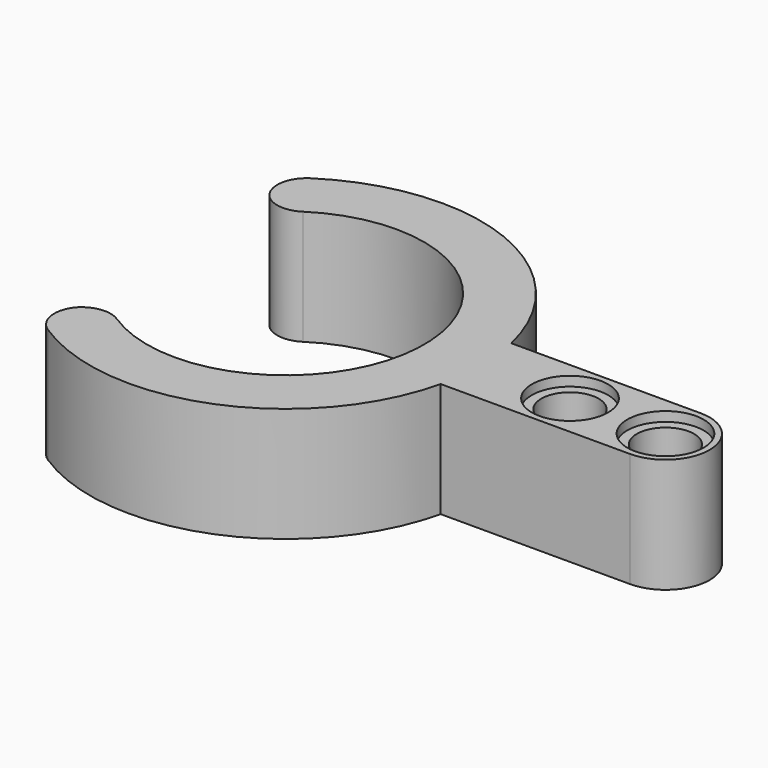
from build123d import *

# Parameters (mm, degrees)
F1_DEPTH    = 9.6
F2_R        = 2.4
F3_DEPTH    = 9.6
F4_T1_DEPTH = 24.0803750693
F4_T3_DEPTH = 20.787199352
F5_R        = 3.2
F6_DEPTH    = 0.8
F7_R        = 3.2
F8_DEPTH    = 0.8


# Not quite as in the source:
# - a fillet or chamfer that OpenCascade refuses, or shapes differently, is made with other operations: its cross-section is extruded or revolved along the edge and cut away or added


with BuildPart() as f1:
    # F0 (on Top) → F1 (new body)
    with BuildSketch(Plane.XY):
        with BuildLine():
            Line((-11.1905737705, 11.9655232935), (-7.9375, 8.4871734989))
            ThreePointArc((-7.9375, 8.4871734989), (11.6205, 0), (-7.9375, -8.4871734989))
            Line((-7.9375, -8.4871734989), (-11.1905737705, -11.9655232935))
            ThreePointArc((-11.1905737705, -11.9655232935), (16.383, 0), (-11.1905737705, 11.9655232935))
        make_face()
    extrude(amount=F1_DEPTH)

    # F2 (on Top) → F3 (join, through all)
    with BuildSketch(Plane.XY):
        with BuildLine():
            Line((31.8347208309, 3.7), (15.9597208309, 3.7))
            ThreePointArc((15.9597208309, 3.7), (16.383, 0), (15.9597208309, -3.7))
            Line((15.9597208309, -3.7), (31.8347208309, -3.7))
            ThreePointArc((31.8347208309, -3.7), (35.5347208309, 0), (31.8347208309, 3.7))
        make_face()
        with Locations((23.8347208309, 0)):
            Circle(F2_R, mode=Mode.SUBTRACT)
        with Locations((31.8347208309, 0)):
            Circle(F2_R, mode=Mode.SUBTRACT)
    extrude(amount=F3_DEPTH)

    # F4: fillet of radius 2.4528409794 on 4 edges, made by hand

    # F4_s2 → F4_t1 (cut)
    with BuildSketch(Plane.XY.offset(-7.2401875346)):
        with BuildLine():
            ThreePointArc((-8.9088227084, 13.7490205815), (-10.0096283387, 11.9889330027), (-9.3664678562, 10.0150976715))
            Line((-9.3664678562, 10.0150976715), (-11.1905737705, 11.9655232935))
            ThreePointArc((-11.1905737705, 11.9655232935), (-10.0891848208, 12.9077898438), (-8.9088227084, 13.7490205815))
        make_face()
        with BuildLine():
            ThreePointArc((-8.9088227084, -13.7490205815), (-10.0096283387, -11.9889330027), (-9.3664678562, -10.0150976715))
            Line((-9.3664678562, -10.0150976715), (-11.1905737705, -11.9655232935))
            ThreePointArc((-11.1905737705, -11.9655232935), (-10.0891848208, -12.9077898438), (-8.9088227084, -13.7490205815))
        make_face()
    extrude(amount=F4_T1_DEPTH, mode=Mode.SUBTRACT)

    # F4_s4 → F4_t3 (cut)
    with BuildSketch(Plane.XY.offset(-5.593599676)):
        with BuildLine():
            ThreePointArc((-9.4658059224, 10.1213149191), (-7.9705260578, 9.3618595516), (-6.3367832056, 9.7406980682))
            ThreePointArc((-6.3367832056, 9.7406980682), (-7.164608937, 9.1490108225), (-7.9375, 8.4871734989))
            Line((-7.9375, 8.4871734989), (-9.4658059224, 10.1213149191))
        make_face()
        with BuildLine():
            ThreePointArc((-9.4658059224, -10.1213149191), (-7.9705260578, -9.3618595516), (-6.3367832056, -9.7406980682))
            ThreePointArc((-6.3367832056, -9.7406980682), (-7.164608937, -9.1490108225), (-7.9375, -8.4871734989))
            Line((-7.9375, -8.4871734989), (-9.4658059224, -10.1213149191))
        make_face()
    extrude(amount=F4_T3_DEPTH, mode=Mode.SUBTRACT)

    # F5 (on face) → F6 (cut)
    with BuildSketch(Plane.XY.offset(9.6)):
        with Locations((23.8347208309, 0)):
            Circle(F5_R)
        with Locations((31.8347208309, 0)):
            Circle(F5_R)
    extrude(amount=-F6_DEPTH, mode=Mode.SUBTRACT)

    # F7 (on face) → F8 (cut)
    with BuildSketch(Plane(origin=(0, 0, 0), x_dir=(1, 0, 0), z_dir=(0, 0, -1))):
        with Locations((23.8347208309, 0)):
            Circle(F7_R)
        with Locations((31.8347208309, 0)):
            Circle(F7_R)
    extrude(amount=-F8_DEPTH, mode=Mode.SUBTRACT)


solid = f1.part
